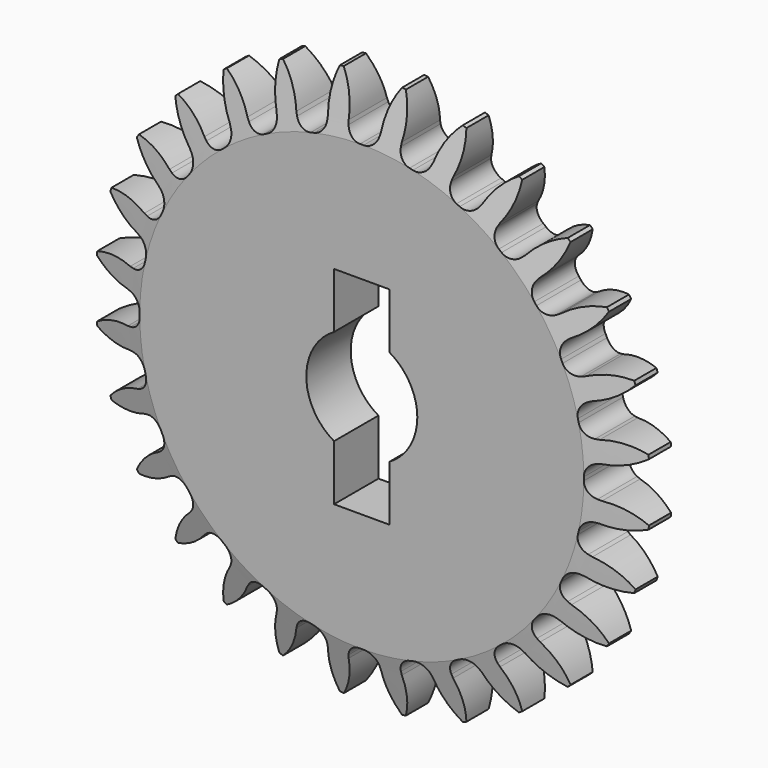
from build123d import *

# Parameters (mm, degrees)
F0_R       = 127
F1_DEPTH   = 25.4
F2_SIZE2   = 6.35
F2_SIZE    = 25.4
F2_2_SIZE2 = 6.35
F2_2_SIZE  = 25.4
F4_DEPTH   = 50.8


# Not quite as in the source:
# - a feature names something its author has since deleted; it is built from what else it names


with BuildPart() as f1:
    # F0 (on Front) → F1 (new body)
    with BuildSketch(Plane.XZ):
        Circle(F0_R)
        with BuildLine():
            ThreePointArc((12.7, 21.9970452561), (21.9970452561, 12.7), (25.4, 0))
            ThreePointArc((25.4, 0), (21.9970452561, -12.7), (12.7, -21.9970452561))
            Line((12.7, -21.9970452561), (12.7, -47.3970452561))
            Line((12.7, -47.3970452561), (-12.7, -47.3970452561))
            Line((-12.7, -47.3970452561), (-12.7, -21.9970452561))
            ThreePointArc((-12.7, -21.9970452561), (-25.4, 0), (-12.7, 21.9970452561))
            Line((-12.7, 21.9970452561), (-12.7, 47.3970452561))
            Line((-12.7, 47.3970452561), (12.7, 47.3970452561))
            Line((12.7, 47.3970452561), (12.7, 21.9970452561))
        make_face(mode=Mode.SUBTRACT)
    extrude(amount=F1_DEPTH)

    # F2
    f2_edges = [f1.edges().sort_by_distance(p)[0] for p in [
        (-127, -25.4, 0),
    ]]
    f2_side = f1.faces().sort_by_distance((-123.407898, -25.4, 0))[0]
    chamfer(f2_edges, length=F2_SIZE, length2=F2_SIZE2, reference=f2_side)

    # F2#2
    f2_2_edges = [f1.edges().sort_by_distance(p)[0] for p in [
        (-127, 0, 0),
    ]]
    f2_2_side = f1.faces().sort_by_distance((-123.407898, 0, 0))[0]
    chamfer(f2_2_edges, length=F2_2_SIZE, length2=F2_2_SIZE2, reference=f2_2_side)

    # F3 (on face) → F4 (cut)
    with BuildSketch(Plane.XZ):
        with BuildLine():
            ThreePointArc((-0.8072971866, 101.5967926229), (0, 101.6), (0.8072971866, 101.5967926229))
            ThreePointArc((0.8072971866, 101.5967926229), (4.8936455243, 103.0441362836), (7.0989916768, 106.776360119))
            Line((7.0989916768, 106.776360119), (7.4142057015, 108.4575018138))
            ThreePointArc((7.4142057015, 108.4575018138), (9.0914439137, 117.8029901103), (13.3318298714, 126.2983068464))
            ThreePointArc((13.3318298714, 126.2983068464), (0, 127), (-13.3318298714, 126.2983068464))
            ThreePointArc((-13.3318298714, 126.2983068464), (-9.0914439137, 117.8029901103), (-7.4142057015, 108.4575018138))
            Line((-7.4142057015, 108.4575018138), (-7.0989916768, 106.776360119))
            ThreePointArc((-7.0989916768, 106.776360119), (-4.8936455243, 103.0441362836), (-0.8072971866, 101.5967926229))
        make_face()
        with BuildLine():
            ThreePointArc((41.1015902587, 120.1651333716), (28.2601586125, 123.8158448471), (15.1064441345, 126.0983558402))
            ThreePointArc((15.1064441345, 126.0983558402), (17.3501289487, 116.8724597877), (16.9057485132, 107.3880617811))
            Line((16.9057485132, 107.3880617811), (16.838970244, 105.6789280992))
            ThreePointArc((16.838970244, 105.6789280992), (18.1585258306, 101.5495432221), (21.8203566207, 99.2291894401))
            ThreePointArc((21.8203566207, 99.2291894401), (22.60812689, 99.0526758777), (23.3944697421, 98.8699083922))
            ThreePointArc((23.3944697421, 98.8699083922), (27.7004290585, 99.3716660771), (30.6809805122, 102.5195795831))
            Line((30.6809805122, 102.5195795831), (31.3623806832, 104.0884298266))
            ThreePointArc((31.3623806832, 104.0884298266), (35.0771338157, 112.8263866063), (41.1015902587, 120.1651333716))
        make_face()
        with BuildLine():
            ThreePointArc((66.8103452851, 108.0063783435), (55.1032348679, 114.4230462236), (42.7872179524, 119.5753067313))
            ThreePointArc((42.7872179524, 119.5753067313), (42.9216938978, 110.0814563144), (40.3779779051, 100.9337359171))
            Line((40.3779779051, 100.9337359171), (39.9325558835, 99.2823133478))
            ThreePointArc((39.9325558835, 99.2823133478), (40.3001528769, 94.9628320295), (43.3538466333, 91.8858203538))
            ThreePointArc((43.3538466333, 91.8858203538), (44.0825878943, 91.5384369789), (44.8085458978, 91.18527411))
            ThreePointArc((44.8085458978, 91.18527411), (49.1181974128, 90.7162855935), (52.7244968721, 93.1220392424))
            Line((52.7244968721, 93.1220392424), (53.7379149396, 94.4999293324))
            ThreePointArc((53.7379149396, 94.4999293324), (59.3039097588, 102.1921969559), (66.8103452851, 108.0063783435))
        make_face()
        with BuildLine():
            ThreePointArc((89.1689506232, 90.43173251), (79.1832048361, 99.2925982734), (68.3224619984, 107.0562524399))
            ThreePointArc((68.3224619984, 107.0562524399), (66.3409858894, 97.7705089614), (61.8254868811, 89.4181710716))
            Line((61.8254868811, 89.4181710716), (61.023756427, 87.9072688383))
            ThreePointArc((61.023756427, 87.9072688383), (60.4209619793, 83.6142879086), (62.7133937457, 79.9349125533))
            ThreePointArc((62.7133937457, 79.9349125533), (63.3465638688, 79.4340786188), (63.9757344581, 78.9282294274))
            ThreePointArc((63.9757344581, 78.9282294274), (68.0729742491, 77.512011752), (72.1241868005, 79.0549710104))
            Line((72.1241868005, 79.0549710104), (73.4188057509, 80.1728077841))
            ThreePointArc((73.4188057509, 80.1728077841), (80.556940035, 86.4336638327), (89.1689506232, 90.43173251))
        make_face()
        with BuildLine():
            ThreePointArc((107.0562524399, 68.3224619984), (99.2925982734, 79.1832048361), (90.43173251, 89.1689506232))
            ThreePointArc((90.43173251, 89.1689506232), (86.4336638327, 80.556940035), (80.1728077841, 73.4188057509))
            Line((80.1728077841, 73.4188057509), (79.0549710104, 72.1241868005))
            ThreePointArc((79.0549710104, 72.1241868005), (77.512011752, 68.0729742491), (78.9282294274, 63.9757344581))
            ThreePointArc((78.9282294274, 63.9757344581), (79.4340786188, 63.3465638688), (79.9349125533, 62.7133937457))
            ThreePointArc((79.9349125533, 62.7133937457), (83.6142879086, 60.4209619793), (87.9072688383, 61.023756427))
            Line((87.9072688383, 61.023756427), (89.4181710716, 61.8254868811))
            ThreePointArc((89.4181710716, 61.8254868811), (97.7705089614, 66.3409858894), (107.0562524399, 68.3224619984))
        make_face()
        with BuildLine():
            ThreePointArc((119.5753067313, 42.7872179524), (114.4230462236, 55.1032348679), (108.0063783435, 66.8103452851))
            ThreePointArc((108.0063783435, 66.8103452851), (102.1921969559, 59.3039097588), (94.4999293324, 53.7379149396))
            Line((94.4999293324, 53.7379149396), (93.1220392424, 52.7244968721))
            ThreePointArc((93.1220392424, 52.7244968721), (90.7162855935, 49.1181974128), (91.18527411, 44.8085458978))
            ThreePointArc((91.18527411, 44.8085458978), (91.5384369789, 44.0825878943), (91.8858203538, 43.3538466333))
            ThreePointArc((91.8858203538, 43.3538466333), (94.9628320295, 40.3001528769), (99.2823133478, 39.9325558835))
            Line((99.2823133478, 39.9325558835), (100.9337359171, 40.3779779051))
            ThreePointArc((100.9337359171, 40.3779779051), (110.0814563144, 42.9216938978), (119.5753067313, 42.7872179524))
        make_face()
        with BuildLine():
            ThreePointArc((126.0983558402, 15.1064441345), (123.8158448471, 28.2601586125), (120.1651333716, 41.1015902587))
            ThreePointArc((120.1651333716, 41.1015902587), (112.8263866063, 35.0771338157), (104.0884298266, 31.3623806832))
            Line((104.0884298266, 31.3623806832), (102.5195795831, 30.6809805122))
            ThreePointArc((102.5195795831, 30.6809805122), (99.3716660771, 27.7004290585), (98.8699083922, 23.3944697421))
            ThreePointArc((98.8699083922, 23.3944697421), (99.0526758777, 22.60812689), (99.2291894401, 21.8203566207))
            ThreePointArc((99.2291894401, 21.8203566207), (101.5495432221, 18.1585258306), (105.6789280992, 16.838970244))
            Line((105.6789280992, 16.838970244), (107.3880617811, 16.9057485132))
            ThreePointArc((107.3880617811, 16.9057485132), (116.8724597877, 17.3501289487), (126.0983558402, 15.1064441345))
        make_face()
        with BuildLine():
            ThreePointArc((127, 0), (126.8244553891, 6.6751415903), (126.2983068464, 13.3318298714))
            ThreePointArc((126.2983068464, 13.3318298714), (117.8029901103, 9.0914439137), (108.4575018138, 7.4142057015))
            Line((108.4575018138, 7.4142057015), (106.776360119, 7.0989916768))
            ThreePointArc((106.776360119, 7.0989916768), (103.0441362836, 4.8936455243), (101.5967926229, 0.8072971866))
            ThreePointArc((101.5967926229, 0.8072971866), (101.6, 0), (101.5967926229, -0.8072971866))
            ThreePointArc((101.5967926229, -0.8072971866), (103.0441362836, -4.8936455243), (106.776360119, -7.0989916768))
            Line((106.776360119, -7.0989916768), (108.4575018138, -7.4142057015))
            ThreePointArc((108.4575018138, -7.4142057015), (117.8029901103, -9.0914439137), (126.2983068464, -13.3318298714))
            ThreePointArc((126.2983068464, -13.3318298714), (126.8244553891, -6.6751415903), (127, 0))
        make_face()
        with BuildLine():
            ThreePointArc((120.1651333716, -41.1015902587), (123.8158448471, -28.2601586125), (126.0983558402, -15.1064441345))
            ThreePointArc((126.0983558402, -15.1064441345), (116.8724597877, -17.3501289487), (107.3880617811, -16.9057485132))
            Line((107.3880617811, -16.9057485132), (105.6789280992, -16.838970244))
            ThreePointArc((105.6789280992, -16.838970244), (101.5495432221, -18.1585258306), (99.2291894401, -21.8203566207))
            ThreePointArc((99.2291894401, -21.8203566207), (99.0526758777, -22.60812689), (98.8699083922, -23.3944697421))
            ThreePointArc((98.8699083922, -23.3944697421), (99.3716660771, -27.7004290585), (102.5195795831, -30.6809805122))
            Line((102.5195795831, -30.6809805122), (104.0884298266, -31.3623806832))
            ThreePointArc((104.0884298266, -31.3623806832), (112.8263866063, -35.0771338157), (120.1651333716, -41.1015902587))
        make_face()
        with BuildLine():
            ThreePointArc((108.0063783435, -66.8103452851), (114.4230462236, -55.1032348679), (119.5753067313, -42.7872179524))
            ThreePointArc((119.5753067313, -42.7872179524), (110.0814563144, -42.9216938978), (100.9337359171, -40.3779779051))
            Line((100.9337359171, -40.3779779051), (99.2823133478, -39.9325558835))
            ThreePointArc((99.2823133478, -39.9325558835), (94.9628320295, -40.3001528769), (91.8858203538, -43.3538466333))
            ThreePointArc((91.8858203538, -43.3538466333), (91.5384369789, -44.0825878943), (91.18527411, -44.8085458978))
            ThreePointArc((91.18527411, -44.8085458978), (90.7162855935, -49.1181974128), (93.1220392424, -52.7244968721))
            Line((93.1220392424, -52.7244968721), (94.4999293324, -53.7379149396))
            ThreePointArc((94.4999293324, -53.7379149396), (102.1921969559, -59.3039097588), (108.0063783435, -66.8103452851))
        make_face()
        with BuildLine():
            ThreePointArc((90.43173251, -89.1689506232), (99.2925982734, -79.1832048361), (107.0562524399, -68.3224619984))
            ThreePointArc((107.0562524399, -68.3224619984), (97.7705089614, -66.3409858894), (89.4181710716, -61.8254868811))
            Line((89.4181710716, -61.8254868811), (87.9072688383, -61.023756427))
            ThreePointArc((87.9072688383, -61.023756427), (83.6142879086, -60.4209619793), (79.9349125533, -62.7133937457))
            ThreePointArc((79.9349125533, -62.7133937457), (79.4340786188, -63.3465638688), (78.9282294274, -63.9757344581))
            ThreePointArc((78.9282294274, -63.9757344581), (77.512011752, -68.0729742491), (79.0549710104, -72.1241868005))
            Line((79.0549710104, -72.1241868005), (80.1728077841, -73.4188057509))
            ThreePointArc((80.1728077841, -73.4188057509), (86.4336638327, -80.556940035), (90.43173251, -89.1689506232))
        make_face()
        with BuildLine():
            ThreePointArc((68.3224619984, -107.0562524399), (79.1832048361, -99.2925982734), (89.1689506232, -90.43173251))
            ThreePointArc((89.1689506232, -90.43173251), (80.556940035, -86.4336638327), (73.4188057509, -80.1728077841))
            Line((73.4188057509, -80.1728077841), (72.1241868005, -79.0549710104))
            ThreePointArc((72.1241868005, -79.0549710104), (68.0729742491, -77.512011752), (63.9757344581, -78.9282294274))
            ThreePointArc((63.9757344581, -78.9282294274), (63.3465638688, -79.4340786188), (62.7133937457, -79.9349125533))
            ThreePointArc((62.7133937457, -79.9349125533), (60.4209619793, -83.6142879086), (61.023756427, -87.9072688383))
            Line((61.023756427, -87.9072688383), (61.8254868811, -89.4181710716))
            ThreePointArc((61.8254868811, -89.4181710716), (66.3409858894, -97.7705089614), (68.3224619984, -107.0562524399))
        make_face()
        with BuildLine():
            ThreePointArc((42.7872179524, -119.5753067313), (55.1032348679, -114.4230462236), (66.8103452851, -108.0063783435))
            ThreePointArc((66.8103452851, -108.0063783435), (59.3039097588, -102.1921969559), (53.7379149396, -94.4999293324))
            Line((53.7379149396, -94.4999293324), (52.7244968721, -93.1220392424))
            ThreePointArc((52.7244968721, -93.1220392424), (49.1181974128, -90.7162855935), (44.8085458978, -91.18527411))
            ThreePointArc((44.8085458978, -91.18527411), (44.0825878943, -91.5384369789), (43.3538466333, -91.8858203538))
            ThreePointArc((43.3538466333, -91.8858203538), (40.3001528769, -94.9628320295), (39.9325558835, -99.2823133478))
            Line((39.9325558835, -99.2823133478), (40.3779779051, -100.9337359171))
            ThreePointArc((40.3779779051, -100.9337359171), (42.9216938978, -110.0814563144), (42.7872179524, -119.5753067313))
        make_face()
        with BuildLine():
            ThreePointArc((15.1064441345, -126.0983558402), (28.2601586125, -123.8158448471), (41.1015902587, -120.1651333716))
            ThreePointArc((41.1015902587, -120.1651333716), (35.0771338157, -112.8263866063), (31.3623806832, -104.0884298266))
            Line((31.3623806832, -104.0884298266), (30.6809805122, -102.5195795831))
            ThreePointArc((30.6809805122, -102.5195795831), (27.7004290585, -99.3716660771), (23.3944697421, -98.8699083922))
            ThreePointArc((23.3944697421, -98.8699083922), (22.60812689, -99.0526758777), (21.8203566207, -99.2291894401))
            ThreePointArc((21.8203566207, -99.2291894401), (18.1585258306, -101.5495432221), (16.838970244, -105.6789280992))
            Line((16.838970244, -105.6789280992), (16.9057485132, -107.3880617811))
            ThreePointArc((16.9057485132, -107.3880617811), (17.3501289487, -116.8724597877), (15.1064441345, -126.0983558402))
        make_face()
        with BuildLine():
            ThreePointArc((-7.4142057015, -108.4575018138), (-9.0914439137, -117.8029901103), (-13.3318298714, -126.2983068464))
            ThreePointArc((-13.3318298714, -126.2983068464), (0, -127), (13.3318298714, -126.2983068464))
            ThreePointArc((13.3318298714, -126.2983068464), (9.0914439137, -117.8029901103), (7.4142057015, -108.4575018138))
            Line((7.4142057015, -108.4575018138), (7.0989916768, -106.776360119))
            ThreePointArc((7.0989916768, -106.776360119), (4.8936455243, -103.0441362836), (0.8072971866, -101.5967926229))
            ThreePointArc((0.8072971866, -101.5967926229), (0, -101.6), (-0.8072971866, -101.5967926229))
            ThreePointArc((-0.8072971866, -101.5967926229), (-4.8936455243, -103.0441362836), (-7.0989916768, -106.776360119))
            Line((-7.0989916768, -106.776360119), (-7.4142057015, -108.4575018138))
        make_face()
        with BuildLine():
            ThreePointArc((-31.3623806832, -104.0884298266), (-35.0771338157, -112.8263866063), (-41.1015902587, -120.1651333716))
            ThreePointArc((-41.1015902587, -120.1651333716), (-28.2601586125, -123.8158448471), (-15.1064441345, -126.0983558402))
            ThreePointArc((-15.1064441345, -126.0983558402), (-17.3501289487, -116.8724597877), (-16.9057485132, -107.3880617811))
            Line((-16.9057485132, -107.3880617811), (-16.838970244, -105.6789280992))
            ThreePointArc((-16.838970244, -105.6789280992), (-18.1585258306, -101.5495432221), (-21.8203566207, -99.2291894401))
            ThreePointArc((-21.8203566207, -99.2291894401), (-22.60812689, -99.0526758777), (-23.3944697421, -98.8699083922))
            ThreePointArc((-23.3944697421, -98.8699083922), (-27.7004290585, -99.3716660771), (-30.6809805122, -102.5195795831))
            Line((-30.6809805122, -102.5195795831), (-31.3623806832, -104.0884298266))
        make_face()
        with BuildLine():
            ThreePointArc((-53.7379149396, -94.4999293324), (-59.3039097588, -102.1921969559), (-66.8103452851, -108.0063783435))
            ThreePointArc((-66.8103452851, -108.0063783435), (-55.1032348679, -114.4230462236), (-42.7872179524, -119.5753067313))
            ThreePointArc((-42.7872179524, -119.5753067313), (-42.9216938978, -110.0814563144), (-40.3779779051, -100.9337359171))
            Line((-40.3779779051, -100.9337359171), (-39.9325558835, -99.2823133478))
            ThreePointArc((-39.9325558835, -99.2823133478), (-40.3001528769, -94.9628320295), (-43.3538466333, -91.8858203538))
            ThreePointArc((-43.3538466333, -91.8858203538), (-44.0825878943, -91.5384369789), (-44.8085458978, -91.18527411))
            ThreePointArc((-44.8085458978, -91.18527411), (-49.1181974128, -90.7162855935), (-52.7244968721, -93.1220392424))
            Line((-52.7244968721, -93.1220392424), (-53.7379149396, -94.4999293324))
        make_face()
        with BuildLine():
            ThreePointArc((-73.4188057509, -80.1728077841), (-80.556940035, -86.4336638327), (-89.1689506232, -90.43173251))
            ThreePointArc((-89.1689506232, -90.43173251), (-79.1832048361, -99.2925982734), (-68.3224619984, -107.0562524399))
            ThreePointArc((-68.3224619984, -107.0562524399), (-66.3409858894, -97.7705089614), (-61.8254868811, -89.4181710716))
            Line((-61.8254868811, -89.4181710716), (-61.023756427, -87.9072688383))
            ThreePointArc((-61.023756427, -87.9072688383), (-60.4209619793, -83.6142879086), (-62.7133937457, -79.9349125533))
            ThreePointArc((-62.7133937457, -79.9349125533), (-63.3465638688, -79.4340786188), (-63.9757344581, -78.9282294274))
            ThreePointArc((-63.9757344581, -78.9282294274), (-68.0729742491, -77.512011752), (-72.1241868005, -79.0549710104))
            Line((-72.1241868005, -79.0549710104), (-73.4188057509, -80.1728077841))
        make_face()
        with BuildLine():
            ThreePointArc((-89.4181710716, -61.8254868811), (-97.7705089614, -66.3409858894), (-107.0562524399, -68.3224619984))
            ThreePointArc((-107.0562524399, -68.3224619984), (-99.2925982734, -79.1832048361), (-90.43173251, -89.1689506232))
            ThreePointArc((-90.43173251, -89.1689506232), (-86.4336638327, -80.556940035), (-80.1728077841, -73.4188057509))
            Line((-80.1728077841, -73.4188057509), (-79.0549710104, -72.1241868005))
            ThreePointArc((-79.0549710104, -72.1241868005), (-77.512011752, -68.0729742491), (-78.9282294274, -63.9757344581))
            ThreePointArc((-78.9282294274, -63.9757344581), (-79.4340786188, -63.3465638688), (-79.9349125533, -62.7133937457))
            ThreePointArc((-79.9349125533, -62.7133937457), (-83.6142879086, -60.4209619793), (-87.9072688383, -61.023756427))
            Line((-87.9072688383, -61.023756427), (-89.4181710716, -61.8254868811))
        make_face()
        with BuildLine():
            ThreePointArc((-100.9337359171, -40.3779779051), (-110.0814563144, -42.9216938978), (-119.5753067313, -42.7872179524))
            ThreePointArc((-119.5753067313, -42.7872179524), (-114.4230462236, -55.1032348679), (-108.0063783435, -66.8103452851))
            ThreePointArc((-108.0063783435, -66.8103452851), (-102.1921969559, -59.3039097588), (-94.4999293324, -53.7379149396))
            Line((-94.4999293324, -53.7379149396), (-93.1220392424, -52.7244968721))
            ThreePointArc((-93.1220392424, -52.7244968721), (-90.7162855935, -49.1181974128), (-91.18527411, -44.8085458978))
            ThreePointArc((-91.18527411, -44.8085458978), (-91.5384369789, -44.0825878943), (-91.8858203538, -43.3538466333))
            ThreePointArc((-91.8858203538, -43.3538466333), (-94.9628320295, -40.3001528769), (-99.2823133478, -39.9325558835))
            Line((-99.2823133478, -39.9325558835), (-100.9337359171, -40.3779779051))
        make_face()
        with BuildLine():
            ThreePointArc((-107.3880617811, -16.9057485132), (-116.8724597877, -17.3501289487), (-126.0983558402, -15.1064441345))
            ThreePointArc((-126.0983558402, -15.1064441345), (-123.8158448471, -28.2601586125), (-120.1651333716, -41.1015902587))
            ThreePointArc((-120.1651333716, -41.1015902587), (-112.8263866063, -35.0771338157), (-104.0884298266, -31.3623806832))
            Line((-104.0884298266, -31.3623806832), (-102.5195795831, -30.6809805122))
            ThreePointArc((-102.5195795831, -30.6809805122), (-99.3716660771, -27.7004290585), (-98.8699083922, -23.3944697421))
            ThreePointArc((-98.8699083922, -23.3944697421), (-99.0526758777, -22.60812689), (-99.2291894401, -21.8203566207))
            ThreePointArc((-99.2291894401, -21.8203566207), (-101.5495432221, -18.1585258306), (-105.6789280992, -16.838970244))
            Line((-105.6789280992, -16.838970244), (-107.3880617811, -16.9057485132))
        make_face()
        with BuildLine():
            ThreePointArc((-108.4575018138, 7.4142057015), (-117.8029901103, 9.0914439137), (-126.2983068464, 13.3318298714))
            ThreePointArc((-126.2983068464, 13.3318298714), (-127, 0), (-126.2983068464, -13.3318298714))
            ThreePointArc((-126.2983068464, -13.3318298714), (-117.8029901103, -9.0914439137), (-108.4575018138, -7.4142057015))
            Line((-108.4575018138, -7.4142057015), (-106.776360119, -7.0989916768))
            ThreePointArc((-106.776360119, -7.0989916768), (-103.0441362836, -4.8936455243), (-101.5967926229, -0.8072971866))
            ThreePointArc((-101.5967926229, -0.8072971866), (-101.6, 0), (-101.5967926229, 0.8072971866))
            ThreePointArc((-101.5967926229, 0.8072971866), (-103.0441362836, 4.8936455243), (-106.776360119, 7.0989916768))
            Line((-106.776360119, 7.0989916768), (-108.4575018138, 7.4142057015))
        make_face()
        with BuildLine():
            ThreePointArc((-104.0884298266, 31.3623806832), (-112.8263866063, 35.0771338157), (-120.1651333716, 41.1015902587))
            ThreePointArc((-120.1651333716, 41.1015902587), (-123.8158448471, 28.2601586125), (-126.0983558402, 15.1064441345))
            ThreePointArc((-126.0983558402, 15.1064441345), (-116.8724597877, 17.3501289487), (-107.3880617811, 16.9057485132))
            Line((-107.3880617811, 16.9057485132), (-105.6789280992, 16.838970244))
            ThreePointArc((-105.6789280992, 16.838970244), (-101.5495432221, 18.1585258306), (-99.2291894401, 21.8203566207))
            ThreePointArc((-99.2291894401, 21.8203566207), (-99.0526758777, 22.60812689), (-98.8699083922, 23.3944697421))
            ThreePointArc((-98.8699083922, 23.3944697421), (-99.3716660771, 27.7004290585), (-102.5195795831, 30.6809805122))
            Line((-102.5195795831, 30.6809805122), (-104.0884298266, 31.3623806832))
        make_face()
        with BuildLine():
            ThreePointArc((-94.4999293324, 53.7379149396), (-102.1921969559, 59.3039097588), (-108.0063783435, 66.8103452851))
            ThreePointArc((-108.0063783435, 66.8103452851), (-114.4230462236, 55.1032348679), (-119.5753067313, 42.7872179524))
            ThreePointArc((-119.5753067313, 42.7872179524), (-110.0814563144, 42.9216938978), (-100.9337359171, 40.3779779051))
            Line((-100.9337359171, 40.3779779051), (-99.2823133478, 39.9325558835))
            ThreePointArc((-99.2823133478, 39.9325558835), (-94.9628320295, 40.3001528769), (-91.8858203538, 43.3538466333))
            ThreePointArc((-91.8858203538, 43.3538466333), (-91.5384369789, 44.0825878943), (-91.18527411, 44.8085458978))
            ThreePointArc((-91.18527411, 44.8085458978), (-90.7162855935, 49.1181974128), (-93.1220392424, 52.7244968721))
            Line((-93.1220392424, 52.7244968721), (-94.4999293324, 53.7379149396))
        make_face()
        with BuildLine():
            ThreePointArc((-80.1728077841, 73.4188057509), (-86.4336638327, 80.556940035), (-90.43173251, 89.1689506232))
            ThreePointArc((-90.43173251, 89.1689506232), (-99.2925982734, 79.1832048361), (-107.0562524399, 68.3224619984))
            ThreePointArc((-107.0562524399, 68.3224619984), (-97.7705089614, 66.3409858894), (-89.4181710716, 61.8254868811))
            Line((-89.4181710716, 61.8254868811), (-87.9072688383, 61.023756427))
            ThreePointArc((-87.9072688383, 61.023756427), (-83.6142879086, 60.4209619793), (-79.9349125533, 62.7133937457))
            ThreePointArc((-79.9349125533, 62.7133937457), (-79.4340786188, 63.3465638688), (-78.9282294274, 63.9757344581))
            ThreePointArc((-78.9282294274, 63.9757344581), (-77.512011752, 68.0729742491), (-79.0549710104, 72.1241868005))
            Line((-79.0549710104, 72.1241868005), (-80.1728077841, 73.4188057509))
        make_face()
        with BuildLine():
            ThreePointArc((-61.8254868811, 89.4181710716), (-66.3409858894, 97.7705089614), (-68.3224619984, 107.0562524399))
            ThreePointArc((-68.3224619984, 107.0562524399), (-79.1832048361, 99.2925982734), (-89.1689506232, 90.43173251))
            ThreePointArc((-89.1689506232, 90.43173251), (-80.556940035, 86.4336638327), (-73.4188057509, 80.1728077841))
            Line((-73.4188057509, 80.1728077841), (-72.1241868005, 79.0549710104))
            ThreePointArc((-72.1241868005, 79.0549710104), (-68.0729742491, 77.512011752), (-63.9757344581, 78.9282294274))
            ThreePointArc((-63.9757344581, 78.9282294274), (-63.3465638688, 79.4340786188), (-62.7133937457, 79.9349125533))
            ThreePointArc((-62.7133937457, 79.9349125533), (-60.4209619793, 83.6142879086), (-61.023756427, 87.9072688383))
            Line((-61.023756427, 87.9072688383), (-61.8254868811, 89.4181710716))
        make_face()
        with BuildLine():
            ThreePointArc((-40.3779779051, 100.9337359171), (-42.9216938978, 110.0814563144), (-42.7872179524, 119.5753067313))
            ThreePointArc((-42.7872179524, 119.5753067313), (-55.1032348679, 114.4230462236), (-66.8103452851, 108.0063783435))
            ThreePointArc((-66.8103452851, 108.0063783435), (-59.3039097588, 102.1921969559), (-53.7379149396, 94.4999293324))
            Line((-53.7379149396, 94.4999293324), (-52.7244968721, 93.1220392424))
            ThreePointArc((-52.7244968721, 93.1220392424), (-49.1181974128, 90.7162855935), (-44.8085458978, 91.18527411))
            ThreePointArc((-44.8085458978, 91.18527411), (-44.0825878943, 91.5384369789), (-43.3538466333, 91.8858203538))
            ThreePointArc((-43.3538466333, 91.8858203538), (-40.3001528769, 94.9628320295), (-39.9325558835, 99.2823133478))
            Line((-39.9325558835, 99.2823133478), (-40.3779779051, 100.9337359171))
        make_face()
        with BuildLine():
            ThreePointArc((-16.9057485132, 107.3880617811), (-17.3501289487, 116.8724597877), (-15.1064441345, 126.0983558402))
            ThreePointArc((-15.1064441345, 126.0983558402), (-28.2601586125, 123.8158448471), (-41.1015902587, 120.1651333716))
            ThreePointArc((-41.1015902587, 120.1651333716), (-35.0771338157, 112.8263866063), (-31.3623806832, 104.0884298266))
            Line((-31.3623806832, 104.0884298266), (-30.6809805122, 102.5195795831))
            ThreePointArc((-30.6809805122, 102.5195795831), (-27.7004290585, 99.3716660771), (-23.3944697421, 98.8699083922))
            ThreePointArc((-23.3944697421, 98.8699083922), (-22.60812689, 99.0526758777), (-21.8203566207, 99.2291894401))
            ThreePointArc((-21.8203566207, 99.2291894401), (-18.1585258306, 101.5495432221), (-16.838970244, 105.6789280992))
            Line((-16.838970244, 105.6789280992), (-16.9057485132, 107.3880617811))
        make_face()
    extrude(amount=F4_DEPTH, mode=Mode.SUBTRACT)


solid = f1.part
